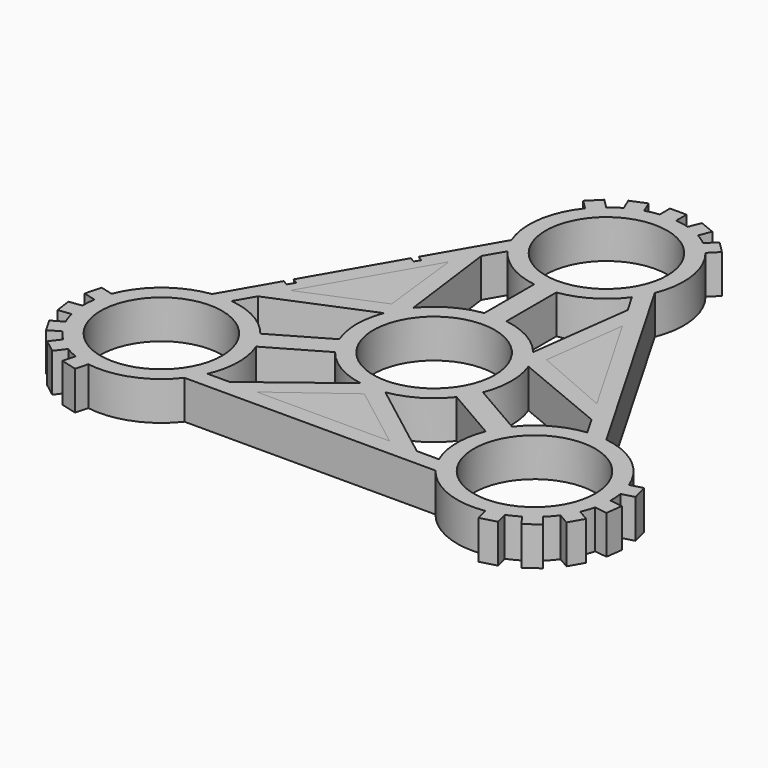
from build123d import *

# Parameters (mm, degrees)
F0_R         = 11
F1_DEPTH     = 7
F2_TEXT_SIZE = 9.7222222222
F3_DEPTH     = 1.1
F5_DEPTH     = 6.8


# Not quite as in the source:
# - Text() gives the source's letters only with a copy of the font that has no kerning and outlines rounded to 1/6400 em; it was checked with that copy


with BuildPart() as f1:
    # F0 (on Top) → F1 (new body)
    with BuildSketch(Plane.XY):
        with BuildLine():
            Line((-12.5511453661, 49.4298250225), (-10.9031700143, 47.7818496707))
            ThreePointArc((-10.9031700143, 47.7818496707), (-13.8516569645, 41.0326335968), (-12.9665216716, 33.720860322))
            Line((-12.9665216716, 33.720860322), (-35.6863825121, -5.6310929947))
            ThreePointArc((-35.6863825121, -5.6310929947), (-42.4611315612, -8.5204299827), (-46.8318806618, -14.4485026212))
            Line((-46.8318806618, -14.4485026212), (-49.0830568571, -13.8453017777))
            Line((-49.0830568571, -13.8453017777), (-49.8595139924, -16.7430792565))
            Line((-49.8595139924, -16.7430792565), (-47.6083377971, -17.3462801001))
            ThreePointArc((-47.6083377971, -17.3462801001), (-47.7450156729, -18.5843561908), (-47.7711084531, -19.8296804116))
            Line((-47.7711084531, -19.8296804116), (-50.0817590332, -20.1338833315))
            Line((-50.0817590332, -20.1338833315), (-49.6901804566, -23.1082179156))
            Line((-49.6901804566, -23.1082179156), (-47.3795298764, -22.8040149957))
            ThreePointArc((-47.3795298764, -22.8040149957), (-47.0320125605, -24.0001525142), (-46.5795541988, -25.1606673479))
            Line((-46.5795541988, -25.1606673479), (-48.5979035591, -26.3259618943))
            Line((-48.5979035591, -26.3259618943), (-47.0979035591, -28.9240381057))
            Line((-47.0979035591, -28.9240381057), (-45.0795541988, -27.7587435592))
            ThreePointArc((-45.0795541988, -27.7587435592), (-44.3007480523, -28.7308414114), (-43.4386212328, -29.6298689945))
            Line((-43.4386212328, -29.6298689945), (-44.8573939794, -31.4788496362))
            Line((-44.8573939794, -31.4788496362), (-42.4773339585, -33.3051339232))
            Line((-42.4773339585, -33.3051339232), (-41.0585612119, -31.4561532815))
            ThreePointArc((-41.0585612119, -31.4561532815), (-39.9670324107, -32.0562183815), (-38.8264881264, -32.5568899142))
            Line((-38.8264881264, -32.5568899142), (-39.4296889699, -34.8080661095))
            Line((-39.4296889699, -34.8080661095), (-36.5319114911, -35.5845232449))
            Line((-36.5319114911, -35.5845232449), (-35.9287106475, -33.3333470495))
            ThreePointArc((-35.9287106475, -33.3333470495), (-28.6094745968, -32.5122036141), (-22.7198608405, -28.0897673273))
            Line((-22.7198608405, -28.0897673273), (22.7198608405, -28.0897673273))
            ThreePointArc((22.7198608405, -28.0897673273), (28.6094745968, -32.5122036141), (35.9287106475, -33.3333470495))
            Line((35.9287106475, -33.3333470495), (36.5319114911, -35.5845232449))
            Line((36.5319114911, -35.5845232449), (39.4296889699, -34.8080661095))
            Line((39.4296889699, -34.8080661095), (38.8264881264, -32.5568899142))
            ThreePointArc((38.8264881264, -32.5568899142), (39.9670324107, -32.0562183815), (41.0585612119, -31.4561532815))
            Line((41.0585612119, -31.4561532815), (42.4773339585, -33.3051339232))
            Line((42.4773339585, -33.3051339232), (44.8573939794, -31.4788496362))
            Line((44.8573939794, -31.4788496362), (43.4386212328, -29.6298689945))
            ThreePointArc((43.4386212328, -29.6298689945), (44.3007480523, -28.7308414114), (45.0795541988, -27.7587435592))
            Line((45.0795541988, -27.7587435592), (47.0979035591, -28.9240381057))
            Line((47.0979035591, -28.9240381057), (48.5979035591, -26.3259618943))
            Line((48.5979035591, -26.3259618943), (46.5795541988, -25.1606673479))
            ThreePointArc((46.5795541988, -25.1606673479), (47.0320125605, -24.0001525142), (47.3795298764, -22.8040149957))
            Line((47.3795298764, -22.8040149957), (49.6901804566, -23.1082179156))
            Line((49.6901804566, -23.1082179156), (50.0817590332, -20.1338833315))
            Line((50.0817590332, -20.1338833315), (47.7711084531, -19.8296804116))
            ThreePointArc((47.7711084531, -19.8296804116), (47.7450156729, -18.5843561908), (47.6083377971, -17.3462801001))
            Line((47.6083377971, -17.3462801001), (49.8595139924, -16.7430792565))
            Line((49.8595139924, -16.7430792565), (49.0830568571, -13.8453017777))
            Line((49.0830568571, -13.8453017777), (46.8318806618, -14.4485026212))
            ThreePointArc((46.8318806618, -14.4485026212), (42.4611315612, -8.5204299827), (35.6863825121, -5.6310929947))
            Line((35.6863825121, -5.6310929947), (12.9665216716, 33.720860322))
            ThreePointArc((12.9665216716, 33.720860322), (13.8516569645, 41.0326335968), (10.9031700143, 47.7818496707))
            Line((10.9031700143, 47.7818496707), (12.5511453661, 49.4298250225))
            Line((12.5511453661, 49.4298250225), (10.4298250225, 51.5511453661))
            Line((10.4298250225, 51.5511453661), (8.7818496707, 49.9031700143))
            ThreePointArc((8.7818496707, 49.9031700143), (7.7779832623, 50.6405745722), (6.7125472412, 51.2858336931))
            Line((6.7125472412, 51.2858336931), (7.6044250747, 53.4390172548))
            Line((7.6044250747, 53.4390172548), (4.8327864772, 54.5870675519))
            Line((4.8327864772, 54.5870675519), (3.9409086437, 52.4338839902))
            ThreePointArc((3.9409086437, 52.4338839902), (2.7312645082, 52.7309939256), (1.5, 52.9194109071))
            Line((1.5, 52.9194109071), (1.5, 55.25))
            Line((1.5, 55.25), (-1.5, 55.25))
            Line((-1.5, 55.25), (-1.5, 52.9194109071))
            ThreePointArc((-1.5, 52.9194109071), (-2.7312645082, 52.7309939256), (-3.9409086437, 52.4338839902))
            Line((-3.9409086437, 52.4338839902), (-4.8327864772, 54.5870675519))
            Line((-4.8327864772, 54.5870675519), (-7.6044250747, 53.4390172548))
            Line((-7.6044250747, 53.4390172548), (-6.7125472412, 51.2858336931))
            ThreePointArc((-6.7125472412, 51.2858336931), (-7.7779832623, 50.6405745722), (-8.7818496707, 49.9031700143))
            Line((-8.7818496707, 49.9031700143), (-10.4298250225, 51.5511453661))
            Line((-10.4298250225, 51.5511453661), (-12.5511453661, 49.4298250225))
        make_face()
        with Locations((-33.7749907476, -19.5)):
            Circle(F0_R, mode=Mode.SUBTRACT)
        Polygon((-12.0180091377, -25.0897673273), (0.1914537595, -16.0356796116), (12.0180091377, -25.0897673273), align=None, mode=Mode.SUBTRACT)
        with BuildLine():
            Line((-20.7749907476, -14.3038475773), (-11, -8.6602540378))
            ThreePointArc((-11, -8.6602540378), (-7.101984242, -12.0649003239), (-2.2333829392, -13.8207091224))
            Line((-2.2333829392, -13.8207091224), (-16.953158703, -25.0897673273))
            Line((-16.953158703, -25.0897673273), (-20.9393177529, -25.0897673273))
            ThreePointArc((-20.9393177529, -25.0897673273), (-19.7766152709, -19.7132698161), (-20.7749907476, -14.3038475773))
        make_face(mode=Mode.SUBTRACT)
        with BuildLine():
            ThreePointArc((-13.085776668, 4.9761881995), (-13.9995022957, -0.1180486089), (-13, -5.1961524227))
            Line((-13, -5.1961524227), (-22.7749907476, -10.8397459622))
            ThreePointArc((-22.7749907476, -10.8397459622), (-26.9605000879, -7.2704163175), (-32.198034757, -5.5890974483))
            Line((-32.198034757, -5.5890974483), (-30.204955232, -2.1369824475))
            Line((-30.204955232, -2.1369824475), (-13.085776668, 4.9761881995))
        make_face(mode=Mode.SUBTRACT)
        with BuildLine():
            ThreePointArc((2.2333829392, -13.8207091224), (7.101984242, -12.0649003239), (11, -8.6602540378))
            Line((11, -8.6602540378), (20.7749907476, -14.3038475773))
            ThreePointArc((20.7749907476, -14.3038475773), (19.7766152709, -19.7132698161), (20.9393177529, -25.0897673273))
            Line((20.9393177529, -25.0897673273), (16.953158703, -25.0897673273))
            Line((16.953158703, -25.0897673273), (2.2333829392, -13.8207091224))
        make_face(mode=Mode.SUBTRACT)
        with Locations((33.7749907476, -19.5)):
            Circle(F0_R, mode=Mode.SUBTRACT)
        with BuildLine():
            Line((22.7749907476, -10.8397459622), (13, -5.1961524227))
            ThreePointArc((13, -5.1961524227), (13.9995022957, -0.1180486089), (13.085776668, 4.9761881995))
            Line((13.085776668, 4.9761881995), (30.204955232, -2.1369824475))
            Line((30.204955232, -2.1369824475), (32.198034757, -5.5890974483))
            ThreePointArc((32.198034757, -5.5890974483), (26.9605000879, -7.2704163175), (22.7749907476, -10.8397459622))
        make_face(mode=Mode.SUBTRACT)
        Circle(F0_R, mode=Mode.SUBTRACT)
        Polygon((-15.7193713117, 22.9527848798), (-13.9830327903, 7.8520359864), (-27.7373804494, 2.1369824475), align=None, mode=Mode.SUBTRACT)
        with BuildLine():
            Line((-2, 25.1435935394), (-2, 13.8564064606))
            ThreePointArc((-2, 13.8564064606), (-6.8975180536, 12.1829489328), (-10.8523937287, 8.844520923))
            Line((-10.8523937287, 8.844520923), (-13.251796529, 27.2267497748))
            Line((-13.251796529, 27.2267497748), (-11.2587170041, 30.6788647756))
            ThreePointArc((-11.2587170041, 30.6788647756), (-7.1838848169, 26.9836861335), (-2, 25.1435935394))
        make_face(mode=Mode.SUBTRACT)
        with BuildLine():
            ThreePointArc((10.8523937287, 8.844520923), (6.8975180536, 12.1829489328), (2, 13.8564064606))
            Line((2, 13.8564064606), (2, 25.1435935394))
            ThreePointArc((2, 25.1435935394), (7.1838848169, 26.9836861335), (11.2587170041, 30.6788647756))
            Line((11.2587170041, 30.6788647756), (13.251796529, 27.2267497748))
            Line((13.251796529, 27.2267497748), (10.8523937287, 8.844520923))
        make_face(mode=Mode.SUBTRACT)
        Polygon((27.7373804494, 2.1369824475), (13.7915790309, 8.1836436252), (15.7193713117, 22.9527848798), align=None, mode=Mode.SUBTRACT)
        with Locations((0, 39)):
            Circle(F0_R, mode=Mode.SUBTRACT)
    extrude(amount=F1_DEPTH)

    # F2 (on face) → F3 (cut)
    with BuildSketch(Plane(origin=(-24.3264520919, 14.0448836637, 0), x_dir=(-0.5, -0.8660254038, 0), z_dir=(-0.8660254038, 0.5, 0))):
        with Locations((-11.8505498394, 0)):
            Text('Corsi', F2_TEXT_SIZE, font='Open Sans', font_style=FontStyle.BOLD, text_align=(TextAlign.LEFT, TextAlign.BOTTOM))
    extrude(amount=-F3_DEPTH, mode=Mode.SUBTRACT)

    # F4 (on face) → F5 (join)
    with BuildSketch(Plane.XY.offset(7)):
        Polygon((27.7373804494, 2.1369824475), (15.7193713117, 22.9527848798), (13.7915790309, 8.1836436252), align=None)
        Polygon((-12.0180091377, -25.0897673273), (12.0180091377, -25.0897673273), (0.1914537595, -16.0356796116), (-11.2587170041, -24.526704264), align=None)
        Polygon((-13.9830327903, 7.8520359864), (-15.7193713117, 22.9527848798), (-27.7373804494, 2.1369824475), align=None)
    extrude(amount=-F5_DEPTH)


solid = f1.part
